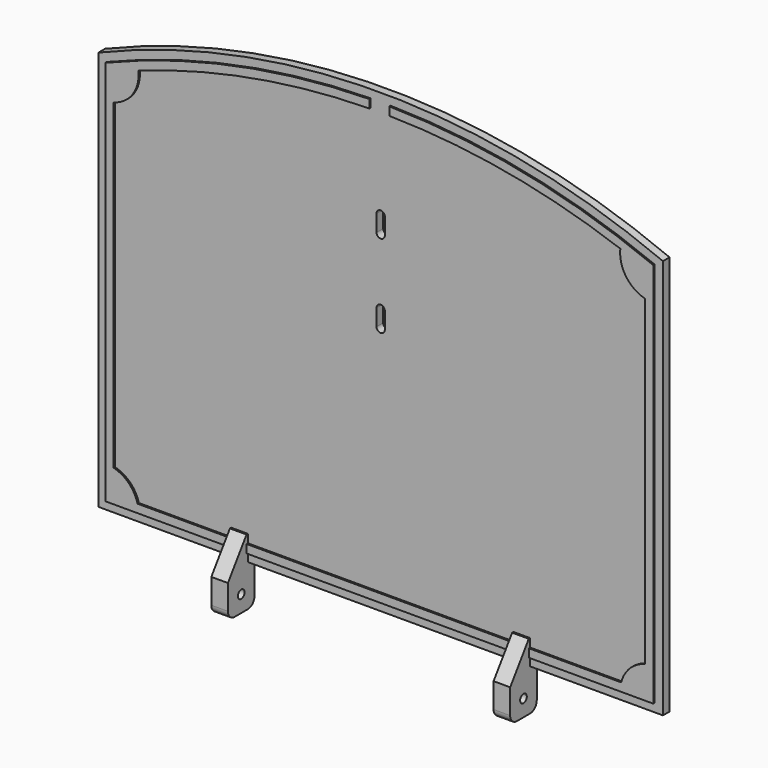
from build123d import *

# Parameters (mm, degrees)
F0_W       = 10
F0_H       = 15
F1_DEPTH   = 5
F3_DEPTH   = 1
F0_H_2     = 25
F4_DEPTH   = 20
F5_SIZE2   = 20
F5_SIZE    = 14
F5_2_SIZE2 = 20
F5_2_SIZE  = 14
F6_R       = 5
F8_D       = 5
F10_DEPTH  = 5


# Not quite as in the source:
# - a feature names something its author has since deleted; it is built from what else it names


with BuildPart() as f1:
    # F0 (on Front) → F1 (new body)
    with BuildSketch(Plane.XZ):
        with BuildLine():
            ThreePointArc((170, 128.3675199291), (0, 162.5), (-170, 128.3675199291))
            Line((-170, 128.3675199291), (-170, -112.5))
            Line((-170, -112.5), (-90, -112.5))
            Line((-90, -112.5), (-90, -97.5))
            Line((-90, -97.5), (-80, -97.5))
            Line((-80, -97.5), (-80, -112.5))
            Line((-80, -112.5), (80, -112.5))
            Line((80, -112.5), (80, -97.5))
            Line((80, -97.5), (90, -97.5))
            Line((90, -97.5), (90, -112.5))
            Line((90, -112.5), (170, -112.5))
            Line((170, -112.5), (170, 128.3675199291))
        make_face()
        with Locations((-85, -105)):
            Rectangle(F0_W, F0_H)
        with Locations((85, -105)):
            Rectangle(F0_W, F0_H)
    extrude(amount=F1_DEPTH)

    # F2 (on face) → F3 (join)
    with BuildSketch(Plane.XZ.offset(5)):
        with BuildLine():
            ThreePointArc((-6, 157.4586583244), (-87.0242594123, 148.7148510214), (-165, 125.0258523247))
            Line((-165, 125.0258523247), (-165, -107.5))
            Line((-165, -107.5), (165, -107.5))
            Line((165, -107.5), (165, 125.0258523247))
            ThreePointArc((165, 125.0258523247), (87.0242594123, 148.7148510214), (6, 157.4586583244))
            Line((6, 157.4586583244), (6, 152.4581780262))
            ThreePointArc((6, 152.4581780262), (76.6048494822, 145.628140857), (145.1290810133, 127.294459524))
            ThreePointArc((145.1290810133, 127.294459524), (148.5184044395, 113.696377148), (160, 105.6609355937))
            Line((160, 105.6609355937), (160, -88.135083269))
            ThreePointArc((160, -88.135083269), (150.8578643763, -93.3578643763), (145.635083269, -102.5))
            Line((145.635083269, -102.5), (-145.635083269, -102.5))
            ThreePointArc((-145.635083269, -102.5), (-150.8578643763, -93.3578643763), (-160, -88.135083269))
            Line((-160, -88.135083269), (-160, 105.6609355937))
            ThreePointArc((-160, 105.6609355937), (-148.5184044395, 113.696377148), (-145.1290810133, 127.294459524))
            ThreePointArc((-145.1290810133, 127.294459524), (-76.6048494822, 145.628140857), (-6, 152.4581780262))
            Line((-6, 152.4581780262), (-6, 157.4586583244))
        make_face()
    extrude(amount=F3_DEPTH)

    # F0 (on Front) → F4 (join)
    with BuildSketch(Plane.XZ):
        with Locations((-85, -125)):
            Rectangle(F0_W, F0_H_2)
        with Locations((85, -125)):
            Rectangle(F0_W, F0_H_2)
        with Locations((85, -105)):
            Rectangle(F0_W, F0_H)
        with Locations((-85, -105)):
            Rectangle(F0_W, F0_H)
    extrude(amount=F4_DEPTH)

    # F5
    f5_edges = [f1.edges().sort_by_distance(p)[0] for p in [
        (85, -20, -97.5),
    ]]
    f5_side = f1.faces().sort_by_distance((85, -12.5, -97.5))[0]
    chamfer(f5_edges, length=F5_SIZE, length2=F5_SIZE2, reference=f5_side)

    # F5#2
    f5_2_edges = [f1.edges().sort_by_distance(p)[0] for p in [
        (-85, -20, -97.5),
    ]]
    f5_2_side = f1.faces().sort_by_distance((-85, -12.5, -97.5))[0]
    chamfer(f5_2_edges, length=F5_2_SIZE, length2=F5_2_SIZE2, reference=f5_2_side)

    # F6
    f6_edges = [f1.edges().sort_by_distance(p)[0] for p in [
        (-85, -20, -137.5),
        (85, -20, -137.5),
        (-85, 0, -137.5),
        (85, 0, -137.5),
    ]]
    fillet(f6_edges, radius=F6_R)

    # F8 (through all)
    with Locations(Plane.YZ.offset(90)):
        with Locations((-10, -127.5)):
            Hole(F8_D / 2)

    # F9 (on face) → F10 (cut)
    with BuildSketch(Plane.XZ.offset(5)):
        with BuildLine():
            Line((2.5, 87.5), (2.5, 97.5))
            ThreePointArc((2.5, 97.5), (0, 100), (-2.5, 97.5))
            Line((-2.5, 97.5), (-2.5, 87.5))
            ThreePointArc((-2.5, 87.5), (0, 85), (2.5, 87.5))
        make_face()
        with BuildLine():
            Line((2.5, 37.5), (2.5, 47.5))
            ThreePointArc((2.5, 47.5), (0, 50), (-2.5, 47.5))
            Line((-2.5, 47.5), (-2.5, 37.5))
            ThreePointArc((-2.5, 37.5), (0, 35), (2.5, 37.5))
        make_face()
    extrude(amount=-F10_DEPTH, mode=Mode.SUBTRACT)


solid = f1.part
